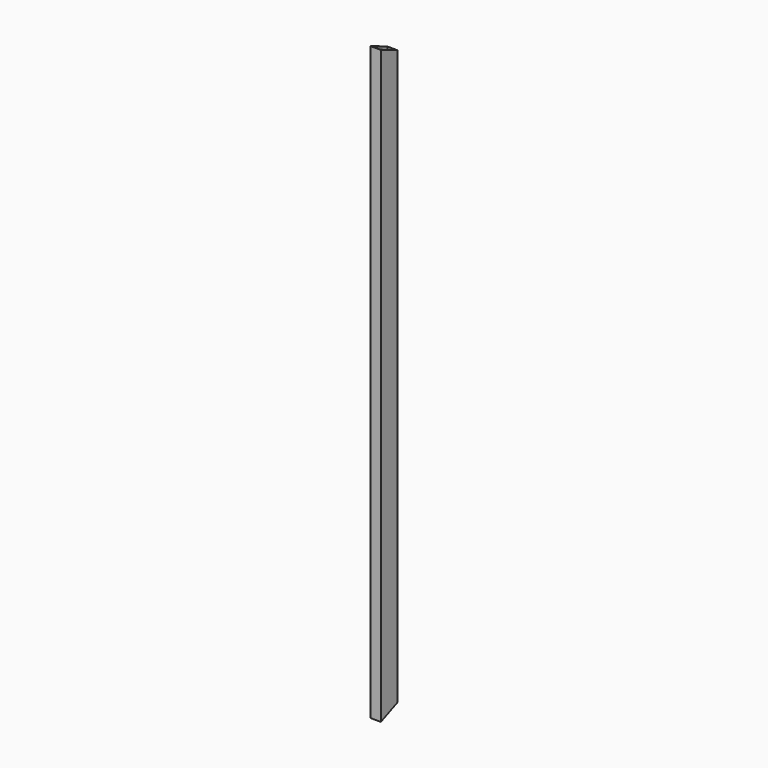
from build123d import *

# Parameters (mm, degrees)
F0_W        = 50
F0_H        = 100
F0_W_2      = 44
F0_H_2      = 94
F1_DEPTH    = 2832
F2_T1_DEPTH = 568.4974851551
F3_T1_DEPTH = 568.4974851551


# Not quite as in the source:
# - a fillet or chamfer that OpenCascade refuses, or shapes differently, is made with other operations: its cross-section is extruded or revolved along the edge and cut away or added


with BuildPart() as f1:
    # F0 (on Top) → F1 (new body)
    with BuildSketch(Plane.XY):
        Rectangle(F0_W, F0_H)
        Rectangle(F0_W_2, F0_H_2, mode=Mode.SUBTRACT)
    extrude(amount=F1_DEPTH)

    # F2: chamfer of 100 x 42 on 1 edges, made by hand

    # F2_s2 → F2_t1 (cut)
    with BuildSketch(Plane.YZ.offset(-284.2487425775)):
        Polygon((50, 2790), (-50, 2832), (50, 2832), align=None)
    extrude(amount=F2_T1_DEPTH, mode=Mode.SUBTRACT)

    # F3: chamfer of 42 x 100 on 1 edges, made by hand

    # F3_s2 → F3_t1 (cut)
    with BuildSketch(Plane.YZ.offset(-284.2487425775)):
        Polygon((-50, 0), (50, 42), (50, 0), align=None)
    extrude(amount=F3_T1_DEPTH, mode=Mode.SUBTRACT)


solid = f1.part
